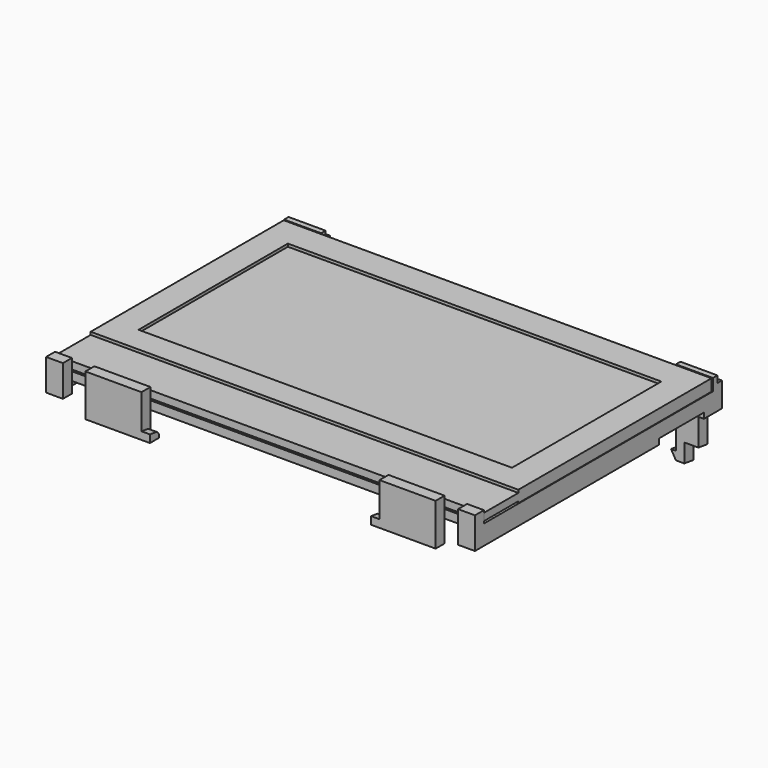
from build123d import *

# Parameters (mm, degrees)
F0_W      = 1.5
F0_H      = 51
F1_DEPTH  = 1.5
F2_DEPTH  = 3.5
F0_W_2    = 10
F0_H_2    = 2
F0_W_3    = 20
F3_DEPTH  = 5.4
F4_DEPTH  = 2.1
F5_W      = 72
F5_H      = 30
F6_DEPTH  = 1
F7_W      = 7.8
F7_H      = 1.3
F8_DEPTH  = 38.1
F9_W      = 66.53
F9_H      = 33.26
F10_DEPTH = 0.5
F12_DEPTH = 1.5
F13_R     = 0.8
F16_W     = 2.5
F16_H     = 1.5
F17_DEPTH = 1.5
F18_W     = 10
F18_H     = 1
F18_W_2   = 1
F18_H_2   = 1.2
F19_DEPTH = 76.401
F20_DEPTH = 1
F21_DEPTH = 7.501


# Not quite as in the source:
# - a pattern or mirror of a feature is missing from the dataset's text; its kind, count and spacing are read off the source's solid


with BuildPart() as f1:
    # F0 (on Top) → F1 (new body)
    with BuildSketch(Plane.XY):
        Polygon((-31.6, 51), (-36.7, 51), (-36.7, 0), (-35.2, 0), (-31.2, 0), (-21.2, 0), (-10, 0), (10, 0), (21.2, 0), (31.2, 0), (35.2, 0), (36.7, 0), (36.7, 51), (31.6, 51), align=None)
        with Locations((-37.45, 25.5)):
            Rectangle(F0_W, F0_H)
        with Locations((37.45, 25.5)):
            Rectangle(F0_W, F0_H)
    extrude(amount=-F1_DEPTH)

    # F0 (on Top) → F2 (join)
    with BuildSketch(Plane.XY):
        Polygon((-36.7, 0), (-38.2, 0), (-38.2, -2), (-35.2, -2), (-35.2, 0), align=None)
        Polygon((38.2, 0), (36.7, 0), (35.2, 0), (35.2, -2), (38.2, -2), align=None)
        with Locations((37.45, 25.5)):
            Rectangle(F0_W, F0_H)
        Polygon((31.6, 53), (31.6, 51), (36.7, 51), (38.2, 51), (38.2, 53), align=None)
        Polygon((-38.2, 53), (-38.2, 51), (-36.7, 51), (-31.6, 51), (-31.6, 53), align=None)
        with Locations((-37.45, 25.5)):
            Rectangle(F0_W, F0_H)
    extrude(amount=-F2_DEPTH)

    # F0 (on Top) → F3 (join)
    with BuildSketch(Plane.XY):
        with Locations((-26.2, -1)):
            Rectangle(F0_W_2, F0_H_2)
        with Locations((0, -1)):
            Rectangle(F0_W_3, F0_H_2)
        with Locations((26.2, -1)):
            Rectangle(F0_W_2, F0_H_2)
    extrude(amount=-F3_DEPTH)

    # F0 (on Top) → F4 (join)
    with BuildSketch(Plane.XY):
        Polygon((-38.2, 53), (-38.2, 51), (-36.7, 51), (-31.6, 51), (-31.6, 53), align=None)
        Polygon((31.6, 53), (31.6, 51), (36.7, 51), (38.2, 51), (38.2, 53), align=None)
        Polygon((-36.7, 0), (-38.2, 0), (-38.2, -2), (-35.2, -2), (-35.2, 0), align=None)
        with Locations((-26.2, -1)):
            Rectangle(F0_W_2, F0_H_2)
        with Locations((26.2, -1)):
            Rectangle(F0_W_2, F0_H_2)
        Polygon((38.2, 0), (36.7, 0), (35.2, 0), (35.2, -2), (38.2, -2), align=None)
        with Locations((0, -1)):
            Rectangle(F0_W_3, F0_H_2)
    extrude(amount=F4_DEPTH)

    # F5 (on face) → F6 (join)
    with BuildSketch(Plane(origin=(0, 0, -1.5), x_dir=(1, 0, 0), z_dir=(0, 0, -1))):
        with Locations((0, -15)):
            Rectangle(F5_W, F5_H)
    extrude(amount=F6_DEPTH)

    # F11 (on face) → F12 (join)
    with BuildSketch(Plane.YZ.offset(-21.2)):
        Polygon((-2, -4.0366079611), (-2, -5.4), (0, -5.4), (0, -4.3176896305), align=None)
    f12 = extrude(amount=F12_DEPTH)

    # F12_copies: F12 across plane
    add(f12.mirror(Plane(origin=(0, 0, 0), x_dir=(0, 0, 1), z_dir=(1, 0, 0))))

    # F13
    f13_edges = [f1.edges().sort_by_distance(p)[0] for p in [
        (20.45, 0, -4.31769),
        (-20.45, 0, -4.31769),
    ]]
    fillet(f13_edges, radius=F13_R)

    # F15: sweep along a path in F11
    with BuildLine(Plane.YZ.offset(-21.2)) as f15_path:
        Line((53, -9.9486642392), (51, -9.6675825698))
    # F14 (on face) → F15 (sweep)
    with BuildSketch(Plane(origin=(0, 53, 0), x_dir=(-1, 0, 0), z_dir=(0, 1, 0))):
        Polygon((35.6, -3.5), (31.6, -3.5), (31.6, -11.7486642392), (30.7339745962, -11.7486642392), (31.6, -13.2486642392), (33.1, -13.2486642392), (33.1, -9.9486642392), (35.6, -9.9486642392), align=None)
    f15 = sweep(path=f15_path.line)

    # F15_copies: F15 across plane
    add(f15.mirror(Plane(origin=(0, 0, 0), x_dir=(0, 0, 1), z_dir=(1, 0, 0))))

    # F16 (on face) → F17 (join)
    with BuildSketch(Plane(origin=(0, 53, 0), x_dir=(-1, 0, 0), z_dir=(0, 1, 0))):
        with Locations((32.85, -2.45)):
            Rectangle(F16_W, F16_H)
    f17 = extrude(amount=F17_DEPTH)

    # F17_copies: F17 across plane
    add(f17.mirror(Plane(origin=(0, 0, 0), x_dir=(0, 0, 1), z_dir=(1, 0, 0))))

    # F18 (on face) → F19 (cut, through all)
    with BuildSketch(Plane(origin=(-38.2, 0, 0), x_dir=(0, -1, 0), z_dir=(-1, 0, 0))):
        with Locations((-44, -3)):
            Rectangle(F18_W, F18_H)
        with Locations((-52.5, 1.5)):
            Rectangle(F18_W_2, F18_H_2)
    extrude(amount=-F19_DEPTH, mode=Mode.SUBTRACT)

    # F20 (cut, through all): a face of the model
    f20_faces = [f1.faces().sort_by_distance(p)[0] for p in [
        (0, 15, -2.5),
    ]]
    extrude(f20_faces, amount=-F20_DEPTH, mode=Mode.SUBTRACT)

    # F21 (cut, through all): a face of the model
    f21_faces = [f1.faces().sort_by_distance(p)[0] for p in [
        (0, -1, -5.4),
    ]]
    extrude(f21_faces, amount=-F21_DEPTH, mode=Mode.SUBTRACT)


with BuildPart() as f8:
    # F7 (on Right) → F8 (new body, symmetric)
    with BuildSketch(Plane.YZ):
        Polygon((50.8, 0), (50.8, 2.1), (7.8, 2.1), (7.8, 1.6), (7.8, 0.3), (7.8, 0), align=None)
        with Locations((3.9, 0.95)):
            Rectangle(F7_W, F7_H)
    extrude(amount=F8_DEPTH, both=True)

    # F9 (on face) → F10 (cut)
    with BuildSketch(Plane.XY.offset(2.1)):
        with Locations((0, 29.05)):
            Rectangle(F9_W, F9_H)
    extrude(amount=-F10_DEPTH, mode=Mode.SUBTRACT)


solid = Compound([f1.part, f8.part])
